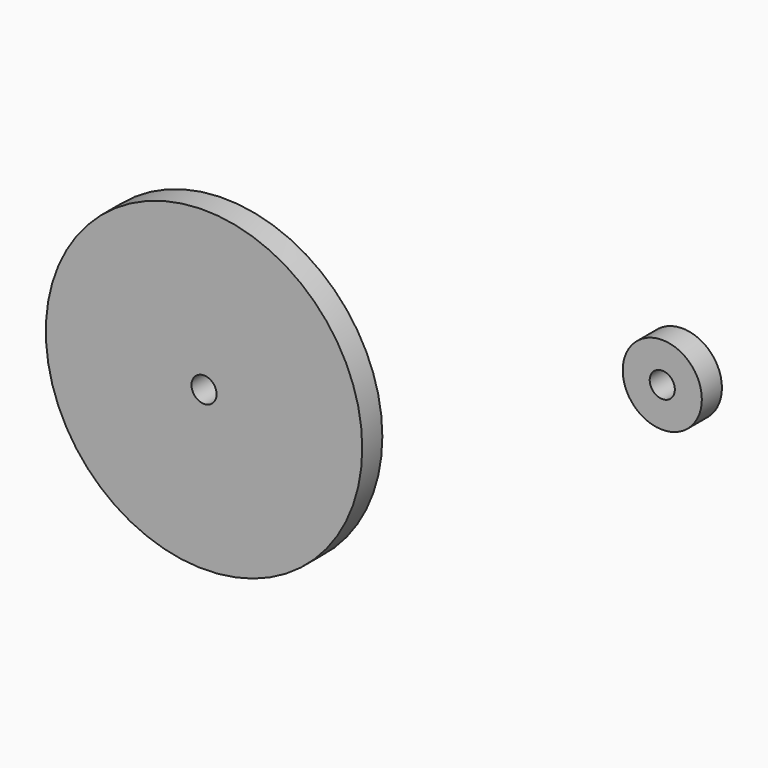
from build123d import *

# Parameters (mm, degrees)
F0_R     = 20
F0_R_2   = 1.5875
F1_DEPTH = 3.175
F2_R     = 5
F2_R_2   = 1.5875
F3_DEPTH = 3.175


# Not quite as in the source:
# - a length typed as a fraction of an inch, garbled in the dataset ("3 / 203.2 mm" for 3/8 in), is restored


with BuildPart() as f1:
    # F0 (on Front) → F1 (new body)
    with BuildSketch(Plane.XZ):
        Circle(F0_R)
        Circle(F0_R_2, mode=Mode.SUBTRACT)
    extrude(amount=F1_DEPTH)


with BuildPart() as f3:
    # F2 (on Front) → F3 (new body)
    with BuildSketch(Plane.XZ):
        with Locations((57.926248759, 19.372086972)):
            Circle(F2_R)
        with Locations((57.926248759, 19.372086972)):
            Circle(F2_R_2, mode=Mode.SUBTRACT)
    extrude(amount=F3_DEPTH)


solid = Compound([f1.part, f3.part])
